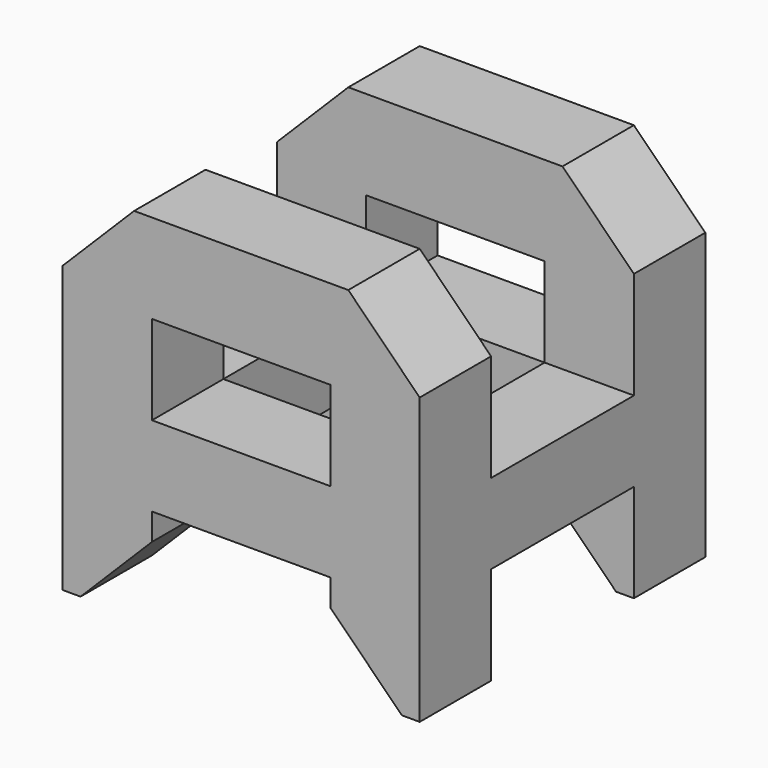
from build123d import *

# Parameters (mm, degrees)
F0_W     = 25.4
F0_H     = 25.4
F1_DEPTH = 25.4
F2_W     = 12.7
F2_H     = 6.985
F2_H_2   = 6.35
F3_DEPTH = 25.401
F4_W     = 12.7
F4_H     = 12.7
F5_DEPTH = 25.401
F6_W     = 12.7
F6_H     = 6.985
F7_DEPTH = 25.401
F8_W     = 12.7
F8_H     = 12.7
F9_DEPTH = 12.701
F10_SIZE = 5.08


with BuildPart() as f1:
    # F0 (on Front) → F1 (new body)
    with BuildSketch(Plane.XZ):
        Rectangle(F0_W, F0_H)
    extrude(amount=F1_DEPTH)

    # F2 (on face) → F3 (cut, through all)
    with BuildSketch(Plane.XZ.offset(25.4)):
        with Locations((0, -9.2075)):
            Rectangle(F2_W, F2_H)
        with Locations((0, 3.175)):
            Rectangle(F2_W, F2_H_2)
    extrude(amount=-F3_DEPTH, mode=Mode.SUBTRACT)

    # F4 (on face) → F5 (cut, through all)
    with BuildSketch(Plane(origin=(-12.7, 0, 0), x_dir=(0, -1, 0), z_dir=(-1, 0, 0))):
        with Locations((12.7, 6.35)):
            Rectangle(F4_W, F4_H)
    extrude(amount=-F5_DEPTH, mode=Mode.SUBTRACT)

    # F6 (on face) → F7 (cut, through all)
    with BuildSketch(Plane.YZ.offset(12.7)):
        with Locations((-12.7, -9.2075)):
            Rectangle(F6_W, F6_H)
    extrude(amount=-F7_DEPTH, mode=Mode.SUBTRACT)

    # F8 (on face) → F9 (cut, through all)
    with BuildSketch(Plane.XY):
        with Locations((0, -12.7)):
            Rectangle(F8_W, F8_H)
    extrude(amount=-F9_DEPTH, mode=Mode.SUBTRACT)

    # F10
    f10_edges = [f1.edges().sort_by_distance(p)[0] for p in [
        (6.35, -22.225, -12.7),
        (6.35, -3.175, -12.7),
        (-6.35, -3.175, -12.7),
        (-6.35, -22.225, -12.7),
        (12.7, -3.175, 12.7),
        (12.7, -22.225, 12.7),
        (-12.7, -22.225, 12.7),
        (-12.7, -3.175, 12.7),
    ]]
    chamfer(f10_edges, length=F10_SIZE)


solid = f1.part
